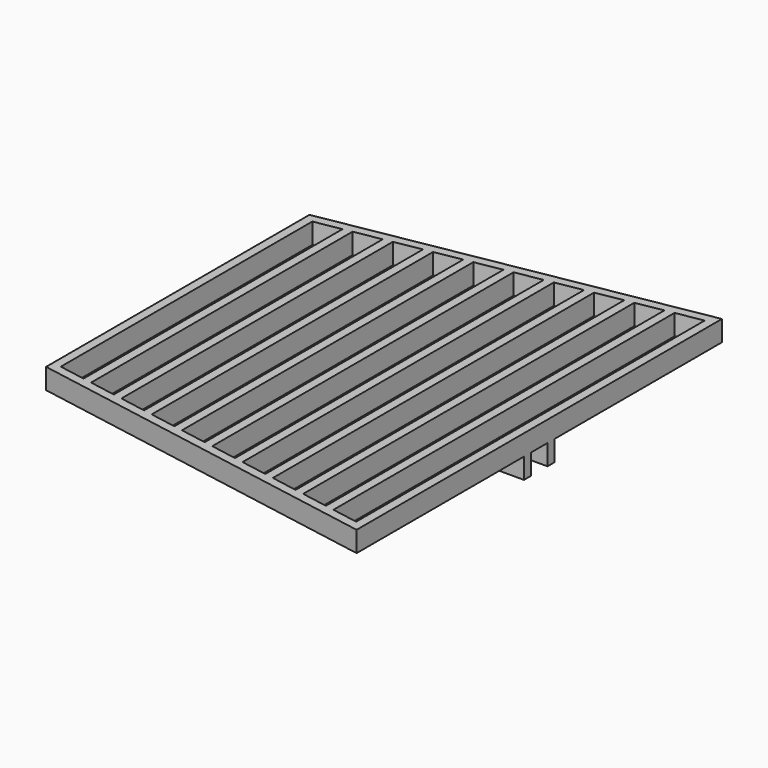
from build123d import *

# Parameters (mm, degrees)
F1_DEPTH = 88.9
F3_W     = 38.1
F3_H     = 88.9
F4_DEPTH = 1562.1


# Not quite as in the source:
# - a feature names something its author has since deleted; it is built from what else it names


with BuildPart() as f1:
    # F0 (on Top) → F1 (new body)
    with BuildSketch(Plane.XY):
        Polygon((535.4871858596, 1118.0772274703), (535.4871858596, 1079.3894735575), (535.4871858596, 406.8772274703), (573.5871858596, 406.8772274703), (573.5871858596, 1086.1075315225), (687.8871858596, 1106.2617054174), (687.8871858597, 406.8772274703), (725.9871858597, 406.8772274703), (725.9871858596, 1112.9797633824), (840.2871858596, 1133.1339372774), (840.2871858596, 406.8772274703), (878.3871858596, 406.8772274703), (878.3871858596, 1139.8519952424), (992.6871858596, 1160.0061691374), (992.6871858596, 406.8772274703), (1030.7871858596, 406.8772274703), (1030.7871858596, 1166.7242271024), (1145.0871858596, 1186.8784009974), (1145.0871858596, 406.8772274703), (1183.1871858596, 406.8772274703), (1183.1871858596, 1193.5964589624), (1297.4871858596, 1213.7506328574), (1297.4871858596, 406.8772274703), (1335.5871858596, 406.8772274703), (1335.5871858596, 1220.4686908224), (1449.8871858596, 1240.6228647173), (1449.8871858596, 406.8772274703), (1487.9871858596, 406.8772274703), (1487.9871858596, 1247.3409226823), (1602.2871858596, 1267.4950965773), (1602.2871858596, 406.8772274703), (1640.3871858596, 406.8772274703), (1640.3871858596, 1274.2131545423), (1754.6871858596, 1294.3673284373), (1754.6871858596, 406.8772274703), (1792.7871858596, 406.8772274703), (1792.7871858596, 1301.0853864023), (1907.0871858596, 1321.2395602973), (1907.0871858596, 406.8772274703), (1945.1871858596, 406.8772274703), (1945.1871858596, 1327.9576182623), (2059.4871858596, 1348.1117921573), (2059.4871858596, 406.8772274703), (2097.5871858597, 406.8772274703), (2097.5871858596, 1354.8298501222), (2097.5871858596, 1393.5176040351), align=None)
    extrude(amount=F1_DEPTH)

    # F2: F1 across face


with BuildPart() as f1_1:
    add(f1.part)
    add(f1.part.mirror(Plane(origin=(554.5371858596, 406.8772274703, 44.45), x_dir=(1, 0, 0), z_dir=(0, -1, 0))))

    # F3 (on face) → F4 (join, through all)
    with BuildSketch(Plane.YZ.offset(2097.5871858597)):
        with Locations((343.3772274703, -44.45)):
            Rectangle(F3_W, F3_H)
        with Locations((470.3772274703, -44.45)):
            Rectangle(F3_W, F3_H)
    extrude(amount=-F4_DEPTH)


solid = f1_1.part
